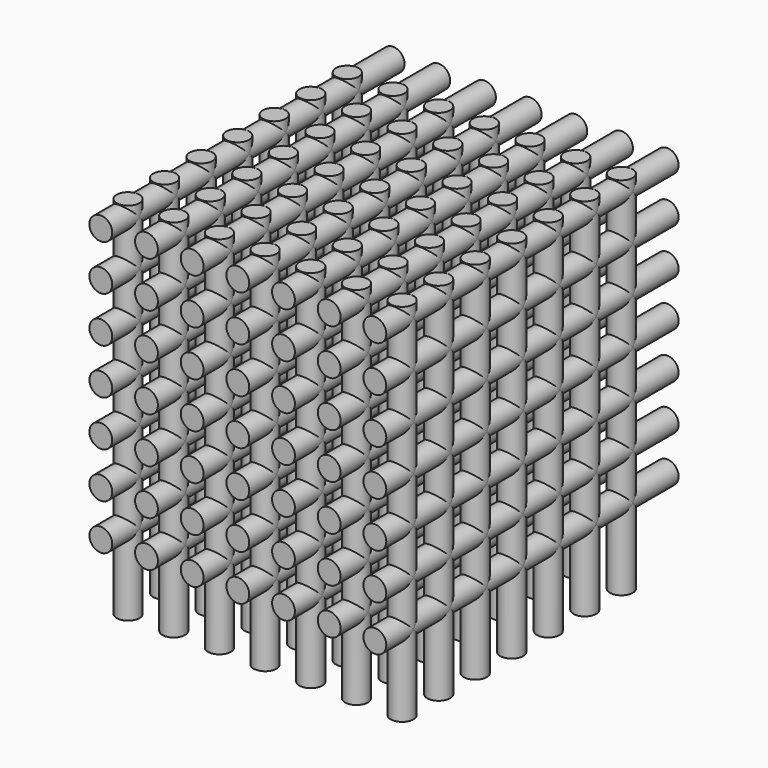
from build123d import *

# Parameters (mm, degrees)
F0_R     = 6.35
F1_DEPTH = 101.6
F2_R     = 6.35
F3_DEPTH = 101.6


with BuildPart() as f1:
    # F0 (on Front) → F1 (new body, symmetric)
    with BuildSketch(Plane.XZ):
        with Locations((-69.8366686702, -57.5505904853)):
            Circle(F0_R)
    extrude(amount=F1_DEPTH, both=True)


with BuildPart() as f1b:
    # F0 (on Front) → F1, piece 2 (new body, symmetric)
    with BuildSketch(Plane.XZ):
        with Locations((-69.8366686702, -32.1505904853)):
            Circle(F0_R)
    extrude(amount=F1_DEPTH, both=True)


with BuildPart() as f1c:
    # F0 (on Front) → F1, piece 3 (new body, symmetric)
    with BuildSketch(Plane.XZ):
        with Locations((-69.8366686702, -6.7505904853)):
            Circle(F0_R)
    extrude(amount=F1_DEPTH, both=True)


with BuildPart() as f1d:
    # F0 (on Front) → F1, piece 4 (new body, symmetric)
    with BuildSketch(Plane.XZ):
        with Locations((-69.8366686702, 18.6494095147)):
            Circle(F0_R)
    extrude(amount=F1_DEPTH, both=True)


with BuildPart() as f1e:
    # F0 (on Front) → F1, piece 5 (new body, symmetric)
    with BuildSketch(Plane.XZ):
        with Locations((-69.8366686702, 44.0494095147)):
            Circle(F0_R)
    extrude(amount=F1_DEPTH, both=True)


with BuildPart() as f1f:
    # F0 (on Front) → F1, piece 6 (new body, symmetric)
    with BuildSketch(Plane.XZ):
        with Locations((-69.8366686702, 69.4494095147)):
            Circle(F0_R)
    extrude(amount=F1_DEPTH, both=True)


with BuildPart() as f1g:
    # F0 (on Front) → F1, piece 7 (new body, symmetric)
    with BuildSketch(Plane.XZ):
        with Locations((-69.8366686702, 94.8494095147)):
            Circle(F0_R)
    extrude(amount=F1_DEPTH, both=True)


with BuildPart() as f1h:
    # F0 (on Front) → F1, piece 8 (new body, symmetric)
    with BuildSketch(Plane.XZ):
        with Locations((-44.4366686702, -57.5505904853)):
            Circle(F0_R)
    extrude(amount=F1_DEPTH, both=True)


with BuildPart() as f1i:
    # F0 (on Front) → F1, piece 9 (new body, symmetric)
    with BuildSketch(Plane.XZ):
        with Locations((-44.4366686702, -32.1505904853)):
            Circle(F0_R)
    extrude(amount=F1_DEPTH, both=True)


with BuildPart() as f1j:
    # F0 (on Front) → F1, piece 10 (new body, symmetric)
    with BuildSketch(Plane.XZ):
        with Locations((-44.4366686702, -6.7505904853)):
            Circle(F0_R)
    extrude(amount=F1_DEPTH, both=True)


with BuildPart() as f1k:
    # F0 (on Front) → F1, piece 11 (new body, symmetric)
    with BuildSketch(Plane.XZ):
        with Locations((-44.4366686702, 18.6494095147)):
            Circle(F0_R)
    extrude(amount=F1_DEPTH, both=True)


with BuildPart() as f1l:
    # F0 (on Front) → F1, piece 12 (new body, symmetric)
    with BuildSketch(Plane.XZ):
        with Locations((-44.4366686702, 44.0494095147)):
            Circle(F0_R)
    extrude(amount=F1_DEPTH, both=True)


with BuildPart() as f1m:
    # F0 (on Front) → F1, piece 13 (new body, symmetric)
    with BuildSketch(Plane.XZ):
        with Locations((-44.4366686702, 69.4494095147)):
            Circle(F0_R)
    extrude(amount=F1_DEPTH, both=True)


with BuildPart() as f1n:
    # F0 (on Front) → F1, piece 14 (new body, symmetric)
    with BuildSketch(Plane.XZ):
        with Locations((-44.4366686702, 94.8494095147)):
            Circle(F0_R)
    extrude(amount=F1_DEPTH, both=True)


with BuildPart() as f1o:
    # F0 (on Front) → F1, piece 15 (new body, symmetric)
    with BuildSketch(Plane.XZ):
        with Locations((-19.0366686702, -57.5505904853)):
            Circle(F0_R)
    extrude(amount=F1_DEPTH, both=True)


with BuildPart() as f1p:
    # F0 (on Front) → F1, piece 16 (new body, symmetric)
    with BuildSketch(Plane.XZ):
        with Locations((-19.0366686702, -32.1505904853)):
            Circle(F0_R)
    extrude(amount=F1_DEPTH, both=True)


with BuildPart() as f1q:
    # F0 (on Front) → F1, piece 17 (new body, symmetric)
    with BuildSketch(Plane.XZ):
        with Locations((-19.0366686702, -6.7505904853)):
            Circle(F0_R)
    extrude(amount=F1_DEPTH, both=True)


with BuildPart() as f1r:
    # F0 (on Front) → F1, piece 18 (new body, symmetric)
    with BuildSketch(Plane.XZ):
        with Locations((-19.0366686702, 18.6494095147)):
            Circle(F0_R)
    extrude(amount=F1_DEPTH, both=True)


with BuildPart() as f1s:
    # F0 (on Front) → F1, piece 19 (new body, symmetric)
    with BuildSketch(Plane.XZ):
        with Locations((-19.0366686702, 44.0494095147)):
            Circle(F0_R)
    extrude(amount=F1_DEPTH, both=True)


with BuildPart() as f1t:
    # F0 (on Front) → F1, piece 20 (new body, symmetric)
    with BuildSketch(Plane.XZ):
        with Locations((-19.0366686702, 69.4494095147)):
            Circle(F0_R)
    extrude(amount=F1_DEPTH, both=True)


with BuildPart() as f1u:
    # F0 (on Front) → F1, piece 21 (new body, symmetric)
    with BuildSketch(Plane.XZ):
        with Locations((-19.0366686702, 94.8494095147)):
            Circle(F0_R)
    extrude(amount=F1_DEPTH, both=True)


with BuildPart() as f1v:
    # F0 (on Front) → F1, piece 22 (new body, symmetric)
    with BuildSketch(Plane.XZ):
        with Locations((6.3633313298, -57.5505904853)):
            Circle(F0_R)
    extrude(amount=F1_DEPTH, both=True)


with BuildPart() as f1w:
    # F0 (on Front) → F1, piece 23 (new body, symmetric)
    with BuildSketch(Plane.XZ):
        with Locations((6.3633313298, -32.1505904853)):
            Circle(F0_R)
    extrude(amount=F1_DEPTH, both=True)


with BuildPart() as f1x:
    # F0 (on Front) → F1, piece 24 (new body, symmetric)
    with BuildSketch(Plane.XZ):
        with Locations((6.3633313298, -6.7505904853)):
            Circle(F0_R)
    extrude(amount=F1_DEPTH, both=True)


with BuildPart() as f1y:
    # F0 (on Front) → F1, piece 25 (new body, symmetric)
    with BuildSketch(Plane.XZ):
        with Locations((6.3633313298, 18.6494095147)):
            Circle(F0_R)
    extrude(amount=F1_DEPTH, both=True)


with BuildPart() as f1z:
    # F0 (on Front) → F1, piece 26 (new body, symmetric)
    with BuildSketch(Plane.XZ):
        with Locations((6.3633313298, 44.0494095147)):
            Circle(F0_R)
    extrude(amount=F1_DEPTH, both=True)


with BuildPart() as f1ba:
    # F0 (on Front) → F1, piece 27 (new body, symmetric)
    with BuildSketch(Plane.XZ):
        with Locations((6.3633313298, 69.4494095147)):
            Circle(F0_R)
    extrude(amount=F1_DEPTH, both=True)


with BuildPart() as f1bb:
    # F0 (on Front) → F1, piece 28 (new body, symmetric)
    with BuildSketch(Plane.XZ):
        with Locations((6.3633313298, 94.8494095147)):
            Circle(F0_R)
    extrude(amount=F1_DEPTH, both=True)


with BuildPart() as f1bc:
    # F0 (on Front) → F1, piece 29 (new body, symmetric)
    with BuildSketch(Plane.XZ):
        with Locations((31.7633313298, -57.5505904853)):
            Circle(F0_R)
    extrude(amount=F1_DEPTH, both=True)


with BuildPart() as f1bd:
    # F0 (on Front) → F1, piece 30 (new body, symmetric)
    with BuildSketch(Plane.XZ):
        with Locations((31.7633313298, -32.1505904853)):
            Circle(F0_R)
    extrude(amount=F1_DEPTH, both=True)


with BuildPart() as f1be:
    # F0 (on Front) → F1, piece 31 (new body, symmetric)
    with BuildSketch(Plane.XZ):
        with Locations((31.7633313298, -6.7505904853)):
            Circle(F0_R)
    extrude(amount=F1_DEPTH, both=True)


with BuildPart() as f1bf:
    # F0 (on Front) → F1, piece 32 (new body, symmetric)
    with BuildSketch(Plane.XZ):
        with Locations((31.7633313298, 18.6494095147)):
            Circle(F0_R)
    extrude(amount=F1_DEPTH, both=True)


with BuildPart() as f1bg:
    # F0 (on Front) → F1, piece 33 (new body, symmetric)
    with BuildSketch(Plane.XZ):
        with Locations((31.7633313298, 44.0494095147)):
            Circle(F0_R)
    extrude(amount=F1_DEPTH, both=True)


with BuildPart() as f1bh:
    # F0 (on Front) → F1, piece 34 (new body, symmetric)
    with BuildSketch(Plane.XZ):
        with Locations((31.7633313298, 69.4494095147)):
            Circle(F0_R)
    extrude(amount=F1_DEPTH, both=True)


with BuildPart() as f1bi:
    # F0 (on Front) → F1, piece 35 (new body, symmetric)
    with BuildSketch(Plane.XZ):
        with Locations((31.7633313298, 94.8494095147)):
            Circle(F0_R)
    extrude(amount=F1_DEPTH, both=True)


with BuildPart() as f1bj:
    # F0 (on Front) → F1, piece 36 (new body, symmetric)
    with BuildSketch(Plane.XZ):
        with Locations((57.1633313298, -57.5505904853)):
            Circle(F0_R)
    extrude(amount=F1_DEPTH, both=True)


with BuildPart() as f1bk:
    # F0 (on Front) → F1, piece 37 (new body, symmetric)
    with BuildSketch(Plane.XZ):
        with Locations((57.1633313298, -32.1505904853)):
            Circle(F0_R)
    extrude(amount=F1_DEPTH, both=True)


with BuildPart() as f1bl:
    # F0 (on Front) → F1, piece 38 (new body, symmetric)
    with BuildSketch(Plane.XZ):
        with Locations((57.1633313298, -6.7505904853)):
            Circle(F0_R)
    extrude(amount=F1_DEPTH, both=True)


with BuildPart() as f1bm:
    # F0 (on Front) → F1, piece 39 (new body, symmetric)
    with BuildSketch(Plane.XZ):
        with Locations((57.1633313298, 18.6494095147)):
            Circle(F0_R)
    extrude(amount=F1_DEPTH, both=True)


with BuildPart() as f1bn:
    # F0 (on Front) → F1, piece 40 (new body, symmetric)
    with BuildSketch(Plane.XZ):
        with Locations((57.1633313298, 44.0494095147)):
            Circle(F0_R)
    extrude(amount=F1_DEPTH, both=True)


with BuildPart() as f1bo:
    # F0 (on Front) → F1, piece 41 (new body, symmetric)
    with BuildSketch(Plane.XZ):
        with Locations((57.1633313298, 69.4494095147)):
            Circle(F0_R)
    extrude(amount=F1_DEPTH, both=True)


with BuildPart() as f1bp:
    # F0 (on Front) → F1, piece 42 (new body, symmetric)
    with BuildSketch(Plane.XZ):
        with Locations((57.1633313298, 94.8494095147)):
            Circle(F0_R)
    extrude(amount=F1_DEPTH, both=True)


with BuildPart() as f1bq:
    # F0 (on Front) → F1, piece 43 (new body, symmetric)
    with BuildSketch(Plane.XZ):
        with Locations((82.5633313298, -57.5505904853)):
            Circle(F0_R)
    extrude(amount=F1_DEPTH, both=True)


with BuildPart() as f1br:
    # F0 (on Front) → F1, piece 44 (new body, symmetric)
    with BuildSketch(Plane.XZ):
        with Locations((82.5633313298, -32.1505904853)):
            Circle(F0_R)
    extrude(amount=F1_DEPTH, both=True)


with BuildPart() as f1bs:
    # F0 (on Front) → F1, piece 45 (new body, symmetric)
    with BuildSketch(Plane.XZ):
        with Locations((82.5633313298, -6.7505904853)):
            Circle(F0_R)
    extrude(amount=F1_DEPTH, both=True)


with BuildPart() as f1bt:
    # F0 (on Front) → F1, piece 46 (new body, symmetric)
    with BuildSketch(Plane.XZ):
        with Locations((82.5633313298, 18.6494095147)):
            Circle(F0_R)
    extrude(amount=F1_DEPTH, both=True)


with BuildPart() as f1bu:
    # F0 (on Front) → F1, piece 47 (new body, symmetric)
    with BuildSketch(Plane.XZ):
        with Locations((82.5633313298, 44.0494095147)):
            Circle(F0_R)
    extrude(amount=F1_DEPTH, both=True)


with BuildPart() as f1bv:
    # F0 (on Front) → F1, piece 48 (new body, symmetric)
    with BuildSketch(Plane.XZ):
        with Locations((82.5633313298, 69.4494095147)):
            Circle(F0_R)
    extrude(amount=F1_DEPTH, both=True)


with BuildPart() as f1bw:
    # F0 (on Front) → F1, piece 49 (new body, symmetric)
    with BuildSketch(Plane.XZ):
        with Locations((82.5633313298, 94.8494095147)):
            Circle(F0_R)
    extrude(amount=F1_DEPTH, both=True)


with BuildPart() as f3:
    # F2 (on Top) → F3 (new body, symmetric)
    with BuildSketch(Plane.XY):
        with Locations((-69.8440269543, -82.6389316045)):
            Circle(F2_R)
    extrude(amount=F3_DEPTH, both=True)


with BuildPart() as f3b:
    # F2 (on Top) → F3, piece 2 (new body, symmetric)
    with BuildSketch(Plane.XY):
        with Locations((-69.8440269543, -57.2389316045)):
            Circle(F2_R)
    extrude(amount=F3_DEPTH, both=True)


with BuildPart() as f3c:
    # F2 (on Top) → F3, piece 3 (new body, symmetric)
    with BuildSketch(Plane.XY):
        with Locations((-69.8440269543, -31.8389316045)):
            Circle(F2_R)
    extrude(amount=F3_DEPTH, both=True)


with BuildPart() as f3d:
    # F2 (on Top) → F3, piece 4 (new body, symmetric)
    with BuildSketch(Plane.XY):
        with Locations((-69.8440269543, -6.4389316045)):
            Circle(F2_R)
    extrude(amount=F3_DEPTH, both=True)


with BuildPart() as f3e:
    # F2 (on Top) → F3, piece 5 (new body, symmetric)
    with BuildSketch(Plane.XY):
        with Locations((-69.8440269543, 18.9610683955)):
            Circle(F2_R)
    extrude(amount=F3_DEPTH, both=True)


with BuildPart() as f3f:
    # F2 (on Top) → F3, piece 6 (new body, symmetric)
    with BuildSketch(Plane.XY):
        with Locations((-69.8440269543, 44.3610683955)):
            Circle(F2_R)
    extrude(amount=F3_DEPTH, both=True)


with BuildPart() as f3g:
    # F2 (on Top) → F3, piece 7 (new body, symmetric)
    with BuildSketch(Plane.XY):
        with Locations((-69.8440269543, 69.7610683955)):
            Circle(F2_R)
    extrude(amount=F3_DEPTH, both=True)


with BuildPart() as f3h:
    # F2 (on Top) → F3, piece 8 (new body, symmetric)
    with BuildSketch(Plane.XY):
        with Locations((-44.4440269543, -82.6389316045)):
            Circle(F2_R)
    extrude(amount=F3_DEPTH, both=True)


with BuildPart() as f3i:
    # F2 (on Top) → F3, piece 9 (new body, symmetric)
    with BuildSketch(Plane.XY):
        with Locations((-44.4440269543, -57.2389316045)):
            Circle(F2_R)
    extrude(amount=F3_DEPTH, both=True)


with BuildPart() as f3j:
    # F2 (on Top) → F3, piece 10 (new body, symmetric)
    with BuildSketch(Plane.XY):
        with Locations((-44.4440269543, -31.8389316045)):
            Circle(F2_R)
    extrude(amount=F3_DEPTH, both=True)


with BuildPart() as f3k:
    # F2 (on Top) → F3, piece 11 (new body, symmetric)
    with BuildSketch(Plane.XY):
        with Locations((-44.4440269543, -6.4389316045)):
            Circle(F2_R)
    extrude(amount=F3_DEPTH, both=True)


with BuildPart() as f3l:
    # F2 (on Top) → F3, piece 12 (new body, symmetric)
    with BuildSketch(Plane.XY):
        with Locations((-44.4440269543, 18.9610683955)):
            Circle(F2_R)
    extrude(amount=F3_DEPTH, both=True)


with BuildPart() as f3m:
    # F2 (on Top) → F3, piece 13 (new body, symmetric)
    with BuildSketch(Plane.XY):
        with Locations((-44.4440269543, 44.3610683955)):
            Circle(F2_R)
    extrude(amount=F3_DEPTH, both=True)


with BuildPart() as f3n:
    # F2 (on Top) → F3, piece 14 (new body, symmetric)
    with BuildSketch(Plane.XY):
        with Locations((-44.4440269543, 69.7610683955)):
            Circle(F2_R)
    extrude(amount=F3_DEPTH, both=True)


with BuildPart() as f3o:
    # F2 (on Top) → F3, piece 15 (new body, symmetric)
    with BuildSketch(Plane.XY):
        with Locations((-19.0440269543, -82.6389316045)):
            Circle(F2_R)
    extrude(amount=F3_DEPTH, both=True)


with BuildPart() as f3p:
    # F2 (on Top) → F3, piece 16 (new body, symmetric)
    with BuildSketch(Plane.XY):
        with Locations((-19.0440269543, -57.2389316045)):
            Circle(F2_R)
    extrude(amount=F3_DEPTH, both=True)


with BuildPart() as f3q:
    # F2 (on Top) → F3, piece 17 (new body, symmetric)
    with BuildSketch(Plane.XY):
        with Locations((-19.0440269543, -31.8389316045)):
            Circle(F2_R)
    extrude(amount=F3_DEPTH, both=True)


with BuildPart() as f3r:
    # F2 (on Top) → F3, piece 18 (new body, symmetric)
    with BuildSketch(Plane.XY):
        with Locations((-19.0440269543, -6.4389316045)):
            Circle(F2_R)
    extrude(amount=F3_DEPTH, both=True)


with BuildPart() as f3s:
    # F2 (on Top) → F3, piece 19 (new body, symmetric)
    with BuildSketch(Plane.XY):
        with Locations((-19.0440269543, 18.9610683955)):
            Circle(F2_R)
    extrude(amount=F3_DEPTH, both=True)


with BuildPart() as f3t:
    # F2 (on Top) → F3, piece 20 (new body, symmetric)
    with BuildSketch(Plane.XY):
        with Locations((-19.0440269543, 44.3610683955)):
            Circle(F2_R)
    extrude(amount=F3_DEPTH, both=True)


with BuildPart() as f3u:
    # F2 (on Top) → F3, piece 21 (new body, symmetric)
    with BuildSketch(Plane.XY):
        with Locations((-19.0440269543, 69.7610683955)):
            Circle(F2_R)
    extrude(amount=F3_DEPTH, both=True)


with BuildPart() as f3v:
    # F2 (on Top) → F3, piece 22 (new body, symmetric)
    with BuildSketch(Plane.XY):
        with Locations((6.3559730457, -82.6389316045)):
            Circle(F2_R)
    extrude(amount=F3_DEPTH, both=True)


with BuildPart() as f3w:
    # F2 (on Top) → F3, piece 23 (new body, symmetric)
    with BuildSketch(Plane.XY):
        with Locations((6.3559730457, -57.2389316045)):
            Circle(F2_R)
    extrude(amount=F3_DEPTH, both=True)


with BuildPart() as f3x:
    # F2 (on Top) → F3, piece 24 (new body, symmetric)
    with BuildSketch(Plane.XY):
        with Locations((6.3559730457, -31.8389316045)):
            Circle(F2_R)
    extrude(amount=F3_DEPTH, both=True)


with BuildPart() as f3y:
    # F2 (on Top) → F3, piece 25 (new body, symmetric)
    with BuildSketch(Plane.XY):
        with Locations((6.3559730457, -6.4389316045)):
            Circle(F2_R)
    extrude(amount=F3_DEPTH, both=True)


with BuildPart() as f3z:
    # F2 (on Top) → F3, piece 26 (new body, symmetric)
    with BuildSketch(Plane.XY):
        with Locations((6.3559730457, 18.9610683955)):
            Circle(F2_R)
    extrude(amount=F3_DEPTH, both=True)


with BuildPart() as f3ba:
    # F2 (on Top) → F3, piece 27 (new body, symmetric)
    with BuildSketch(Plane.XY):
        with Locations((6.3559730457, 44.3610683955)):
            Circle(F2_R)
    extrude(amount=F3_DEPTH, both=True)


with BuildPart() as f3bb:
    # F2 (on Top) → F3, piece 28 (new body, symmetric)
    with BuildSketch(Plane.XY):
        with Locations((6.3559730457, 69.7610683955)):
            Circle(F2_R)
    extrude(amount=F3_DEPTH, both=True)


with BuildPart() as f3bc:
    # F2 (on Top) → F3, piece 29 (new body, symmetric)
    with BuildSketch(Plane.XY):
        with Locations((31.7559730457, -82.6389316045)):
            Circle(F2_R)
    extrude(amount=F3_DEPTH, both=True)


with BuildPart() as f3bd:
    # F2 (on Top) → F3, piece 30 (new body, symmetric)
    with BuildSketch(Plane.XY):
        with Locations((31.7559730457, -57.2389316045)):
            Circle(F2_R)
    extrude(amount=F3_DEPTH, both=True)


with BuildPart() as f3be:
    # F2 (on Top) → F3, piece 31 (new body, symmetric)
    with BuildSketch(Plane.XY):
        with Locations((31.7559730457, -31.8389316045)):
            Circle(F2_R)
    extrude(amount=F3_DEPTH, both=True)


with BuildPart() as f3bf:
    # F2 (on Top) → F3, piece 32 (new body, symmetric)
    with BuildSketch(Plane.XY):
        with Locations((31.7559730457, -6.4389316045)):
            Circle(F2_R)
    extrude(amount=F3_DEPTH, both=True)


with BuildPart() as f3bg:
    # F2 (on Top) → F3, piece 33 (new body, symmetric)
    with BuildSketch(Plane.XY):
        with Locations((31.7559730457, 18.9610683955)):
            Circle(F2_R)
    extrude(amount=F3_DEPTH, both=True)


with BuildPart() as f3bh:
    # F2 (on Top) → F3, piece 34 (new body, symmetric)
    with BuildSketch(Plane.XY):
        with Locations((31.7559730457, 44.3610683955)):
            Circle(F2_R)
    extrude(amount=F3_DEPTH, both=True)


with BuildPart() as f3bi:
    # F2 (on Top) → F3, piece 35 (new body, symmetric)
    with BuildSketch(Plane.XY):
        with Locations((31.7559730457, 69.7610683955)):
            Circle(F2_R)
    extrude(amount=F3_DEPTH, both=True)


with BuildPart() as f3bj:
    # F2 (on Top) → F3, piece 36 (new body, symmetric)
    with BuildSketch(Plane.XY):
        with Locations((57.1559730457, -82.6389316045)):
            Circle(F2_R)
    extrude(amount=F3_DEPTH, both=True)


with BuildPart() as f3bk:
    # F2 (on Top) → F3, piece 37 (new body, symmetric)
    with BuildSketch(Plane.XY):
        with Locations((57.1559730457, -57.2389316045)):
            Circle(F2_R)
    extrude(amount=F3_DEPTH, both=True)


with BuildPart() as f3bl:
    # F2 (on Top) → F3, piece 38 (new body, symmetric)
    with BuildSketch(Plane.XY):
        with Locations((57.1559730457, -31.8389316045)):
            Circle(F2_R)
    extrude(amount=F3_DEPTH, both=True)


with BuildPart() as f3bm:
    # F2 (on Top) → F3, piece 39 (new body, symmetric)
    with BuildSketch(Plane.XY):
        with Locations((57.1559730457, -6.4389316045)):
            Circle(F2_R)
    extrude(amount=F3_DEPTH, both=True)


with BuildPart() as f3bn:
    # F2 (on Top) → F3, piece 40 (new body, symmetric)
    with BuildSketch(Plane.XY):
        with Locations((57.1559730457, 18.9610683955)):
            Circle(F2_R)
    extrude(amount=F3_DEPTH, both=True)


with BuildPart() as f3bo:
    # F2 (on Top) → F3, piece 41 (new body, symmetric)
    with BuildSketch(Plane.XY):
        with Locations((57.1559730457, 44.3610683955)):
            Circle(F2_R)
    extrude(amount=F3_DEPTH, both=True)


with BuildPart() as f3bp:
    # F2 (on Top) → F3, piece 42 (new body, symmetric)
    with BuildSketch(Plane.XY):
        with Locations((57.1559730457, 69.7610683955)):
            Circle(F2_R)
    extrude(amount=F3_DEPTH, both=True)


with BuildPart() as f3bq:
    # F2 (on Top) → F3, piece 43 (new body, symmetric)
    with BuildSketch(Plane.XY):
        with Locations((82.5559730457, -82.6389316045)):
            Circle(F2_R)
    extrude(amount=F3_DEPTH, both=True)


with BuildPart() as f3br:
    # F2 (on Top) → F3, piece 44 (new body, symmetric)
    with BuildSketch(Plane.XY):
        with Locations((82.5559730457, -57.2389316045)):
            Circle(F2_R)
    extrude(amount=F3_DEPTH, both=True)


with BuildPart() as f3bs:
    # F2 (on Top) → F3, piece 45 (new body, symmetric)
    with BuildSketch(Plane.XY):
        with Locations((82.5559730457, -31.8389316045)):
            Circle(F2_R)
    extrude(amount=F3_DEPTH, both=True)


with BuildPart() as f3bt:
    # F2 (on Top) → F3, piece 46 (new body, symmetric)
    with BuildSketch(Plane.XY):
        with Locations((82.5559730457, -6.4389316045)):
            Circle(F2_R)
    extrude(amount=F3_DEPTH, both=True)


with BuildPart() as f3bu:
    # F2 (on Top) → F3, piece 47 (new body, symmetric)
    with BuildSketch(Plane.XY):
        with Locations((82.5559730457, 18.9610683955)):
            Circle(F2_R)
    extrude(amount=F3_DEPTH, both=True)


with BuildPart() as f3bv:
    # F2 (on Top) → F3, piece 48 (new body, symmetric)
    with BuildSketch(Plane.XY):
        with Locations((82.5559730457, 44.3610683955)):
            Circle(F2_R)
    extrude(amount=F3_DEPTH, both=True)


with BuildPart() as f3bw:
    # F2 (on Top) → F3, piece 49 (new body, symmetric)
    with BuildSketch(Plane.XY):
        with Locations((82.5559730457, 69.7610683955)):
            Circle(F2_R)
    extrude(amount=F3_DEPTH, both=True)


solid = Compound([f1.part, f1b.part, f1c.part, f1d.part, f1e.part, f1f.part, f1g.part, f1h.part, f1i.part, f1j.part, f1k.part, f1l.part, f1m.part, f1n.part, f1o.part, f1p.part, f1q.part, f1r.part, f1s.part, f1t.part, f1u.part, f1v.part, f1w.part, f1x.part, f1y.part, f1z.part, f1ba.part, f1bb.part, f1bc.part, f1bd.part, f1be.part, f1bf.part, f1bg.part, f1bh.part, f1bi.part, f1bj.part, f1bk.part, f1bl.part, f1bm.part, f1bn.part, f1bo.part, f1bp.part, f1bq.part, f1br.part, f1bs.part, f1bt.part, f1bu.part, f1bv.part, f1bw.part, f3.part, f3b.part, f3c.part, f3d.part, f3e.part, f3f.part, f3g.part, f3h.part, f3i.part, f3j.part, f3k.part, f3l.part, f3m.part, f3n.part, f3o.part, f3p.part, f3q.part, f3r.part, f3s.part, f3t.part, f3u.part, f3v.part, f3w.part, f3x.part, f3y.part, f3z.part, f3ba.part, f3bb.part, f3bc.part, f3bd.part, f3be.part, f3bf.part, f3bg.part, f3bh.part, f3bi.part, f3bj.part, f3bk.part, f3bl.part, f3bm.part, f3bn.part, f3bo.part, f3bp.part, f3bq.part, f3br.part, f3bs.part, f3bt.part, f3bu.part, f3bv.part, f3bw.part])
